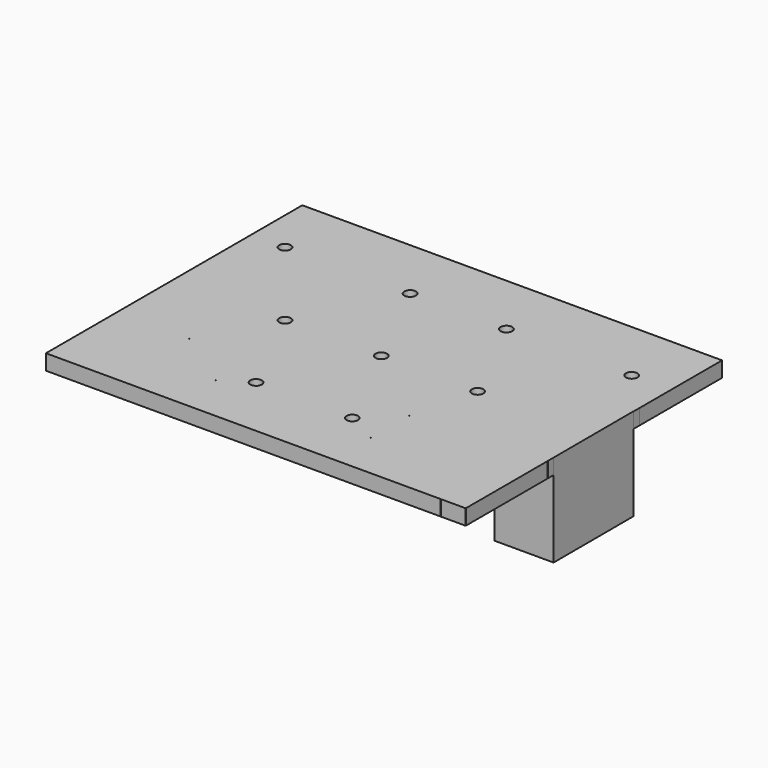
from build123d import *

# Parameters (mm, degrees)
F1_DEPTH = 2.54
F3_DEPTH = 12.7
F4_DEPTH = 2.54


# Not quite as in the source:
# - a feature names something its author has since deleted; it is built from what else it names


with BuildPart() as f1:
    # F0 (on Top) → F1 (new body)
    with BuildSketch(Plane.XY):
        with BuildLine():
            ThreePointArc((24.89835, -8.3058), (24.9076493597, -8.2833493597), (24.9301, -8.27405))
            Line((24.9301, -8.27405), (24.9301, 8.14705))
            ThreePointArc((24.9301, 8.14705), (24.9076493597, 8.1563493597), (24.89835, 8.1788))
            ThreePointArc((24.89835, 8.1788), (24.9301, 8.21055), (24.96185, 8.1788))
            Line((24.96185, 8.1788), (34.57575, 8.1788))
            ThreePointArc((34.57575, 8.1788), (34.5850493597, 8.2012506403), (34.6075, 8.21055))
            Line((34.6075, 8.21055), (34.6075, 9.36625))
            ThreePointArc((34.6075, 9.36625), (34.5850493597, 9.3755493597), (34.57575, 9.398))
            ThreePointArc((34.57575, 9.398), (34.5850493597, 9.4204506403), (34.6075, 9.42975))
            Line((34.6075, 9.42975), (34.6075, 26.38425))
            ThreePointArc((34.6075, 26.38425), (34.5850493597, 26.3935493597), (34.57575, 26.416))
            Line((34.57575, 26.416), (-34.57575, 26.416))
            ThreePointArc((-34.57575, 26.416), (-34.5850493597, 26.3935493597), (-34.6075, 26.38425))
            Line((-34.6075, 26.38425), (-34.6075, -26.38425))
            ThreePointArc((-34.6075, -26.38425), (-34.5850493597, -26.3935493597), (-34.57575, -26.416))
            Line((-34.57575, -26.416), (30.48635, -26.416))
            ThreePointArc((30.48635, -26.416), (30.5181, -26.38425), (30.54985, -26.416))
            Line((30.54985, -26.416), (34.57575, -26.416))
            ThreePointArc((34.57575, -26.416), (34.5850493597, -26.3935493597), (34.6075, -26.38425))
            Line((34.6075, -26.38425), (34.6075, -9.55675))
            ThreePointArc((34.6075, -9.55675), (34.5850493597, -9.5474506403), (34.57575, -9.525))
            ThreePointArc((34.57575, -9.525), (34.5850493597, -9.5025493597), (34.6075, -9.49325))
            Line((34.6075, -9.49325), (34.6075, -8.33755))
            ThreePointArc((34.6075, -8.33755), (34.5850493597, -8.3282506403), (34.57575, -8.3058))
            Line((34.57575, -8.3058), (24.96185, -8.3058))
            ThreePointArc((24.96185, -8.3058), (24.9301, -8.33755), (24.89835, -8.3058))
        make_face()
        with BuildLine():
            Line((-12.8397, -11.79195), (-12.8397, -18.61185))
            ThreePointArc((-12.8397, -18.61185), (-12.8172493597, -18.6211493597), (-12.80795, -18.6436))
            ThreePointArc((-12.80795, -18.6436), (-12.8397, -18.67535), (-12.87145, -18.6436))
            Line((-12.87145, -18.6436), (-22.68855, -18.6436))
            ThreePointArc((-22.68855, -18.6436), (-22.7203, -18.67535), (-22.75205, -18.6436))
            ThreePointArc((-22.75205, -18.6436), (-22.7427506403, -18.6211493597), (-22.7203, -18.61185))
            Line((-22.7203, -18.61185), (-22.7203, -11.79195))
            ThreePointArc((-22.7203, -11.79195), (-22.7427506403, -11.7826506403), (-22.75205, -11.7602))
            ThreePointArc((-22.75205, -11.7602), (-22.7203, -11.72845), (-22.68855, -11.7602))
            Line((-22.68855, -11.7602), (-12.87145, -11.7602))
            ThreePointArc((-12.87145, -11.7602), (-12.8397, -11.72845), (-12.80795, -11.7602))
            ThreePointArc((-12.80795, -11.7602), (-12.8172493597, -11.7826506403), (-12.8397, -11.79195))
        make_face(mode=Mode.SUBTRACT)
        with BuildLine():
            ThreePointArc((-12.21105, -24.6126), (-12.2017506403, -24.5901493597), (-12.1793, -24.58085))
            Line((-12.1793, -24.58085), (-12.1793, -20.91055))
            ThreePointArc((-12.1793, -20.91055), (-12.2017506403, -20.9012506403), (-12.21105, -20.8788))
            ThreePointArc((-12.21105, -20.8788), (-12.1793, -20.84705), (-12.14755, -20.8788))
            Line((-12.14755, -20.8788), (9.22655, -20.8788))
            ThreePointArc((9.22655, -20.8788), (9.2583, -20.84705), (9.29005, -20.8788))
            ThreePointArc((9.29005, -20.8788), (9.2807506403, -20.9012506403), (9.2583, -20.91055))
            Line((9.2583, -20.91055), (9.2583, -24.58085))
            ThreePointArc((9.2583, -24.58085), (9.2807506403, -24.5901493597), (9.29005, -24.6126))
            ThreePointArc((9.29005, -24.6126), (9.2583, -24.64435), (9.22655, -24.6126))
            Line((9.22655, -24.6126), (-12.14755, -24.6126))
            ThreePointArc((-12.14755, -24.6126), (-12.1793, -24.64435), (-12.21105, -24.6126))
        make_face(mode=Mode.SUBTRACT)
        with BuildLine():
            ThreePointArc((-7.4422, -15.875), (-8.3947, -16.8275), (-9.3472, -15.875))
            ThreePointArc((-9.3472, -15.875), (-8.3947, -14.9225), (-7.4422, -15.875))
        make_face(mode=Mode.SUBTRACT)
        with BuildLine():
            ThreePointArc((8.4328, -15.875), (7.4803, -16.8275), (6.5278, -15.875))
            ThreePointArc((6.5278, -15.875), (7.4803, -14.9225), (8.4328, -15.875))
        make_face(mode=Mode.SUBTRACT)
        with BuildLine():
            ThreePointArc((12.75715, -18.669), (12.7664493597, -18.6465493597), (12.7889, -18.63725))
            Line((12.7889, -18.63725), (12.7889, -10.82675))
            ThreePointArc((12.7889, -10.82675), (12.7664493597, -10.8174506403), (12.75715, -10.795))
            ThreePointArc((12.75715, -10.795), (12.7889, -10.76325), (12.82065, -10.795))
            Line((12.82065, -10.795), (18.90395, -10.795))
            ThreePointArc((18.90395, -10.795), (18.9357, -10.76325), (18.96745, -10.795))
            ThreePointArc((18.96745, -10.795), (18.9581506403, -10.8174506403), (18.9357, -10.82675))
            Line((18.9357, -10.82675), (18.9357, -18.63725))
            ThreePointArc((18.9357, -18.63725), (18.9581506403, -18.6465493597), (18.96745, -18.669))
            ThreePointArc((18.96745, -18.669), (18.9357, -18.70075), (18.90395, -18.669))
            Line((18.90395, -18.669), (12.82065, -18.669))
            ThreePointArc((12.82065, -18.669), (12.7889, -18.70075), (12.75715, -18.669))
        make_face(mode=Mode.SUBTRACT)
        with BuildLine():
            ThreePointArc((-15.367, 0), (-16.3195, -0.9525), (-17.272, 0))
            ThreePointArc((-17.272, 0), (-16.3195, 0.9525), (-15.367, 0))
        make_face(mode=Mode.SUBTRACT)
        with BuildLine():
            ThreePointArc((0.508, 0), (-0.4445, -0.9525), (-1.397, 0))
            ThreePointArc((-1.397, 0), (-0.4445, 0.9525), (0.508, 0))
        make_face(mode=Mode.SUBTRACT)
        with BuildLine():
            ThreePointArc((-28.067, 15.875), (-29.0195, 14.9225), (-29.972, 15.875))
            ThreePointArc((-29.972, 15.875), (-29.0195, 16.8275), (-28.067, 15.875))
        make_face(mode=Mode.SUBTRACT)
        with BuildLine():
            ThreePointArc((-7.4422, 15.875), (-8.3947, 14.9225), (-9.3472, 15.875))
            ThreePointArc((-9.3472, 15.875), (-8.3947, 16.8275), (-7.4422, 15.875))
        make_face(mode=Mode.SUBTRACT)
        with BuildLine():
            ThreePointArc((16.383, 0), (15.4305, -0.9525), (14.478, 0))
            ThreePointArc((14.478, 0), (15.4305, 0.9525), (16.383, 0))
        make_face(mode=Mode.SUBTRACT)
        with BuildLine():
            ThreePointArc((8.4328, 15.875), (7.4803, 14.9225), (6.5278, 15.875))
            ThreePointArc((6.5278, 15.875), (7.4803, 16.8275), (8.4328, 15.875))
        make_face(mode=Mode.SUBTRACT)
        with BuildLine():
            ThreePointArc((29.083, 15.875), (28.1305, 14.9225), (27.178, 15.875))
            ThreePointArc((27.178, 15.875), (28.1305, 16.8275), (29.083, 15.875))
        make_face(mode=Mode.SUBTRACT)
        with BuildLine():
            Line((12.7889, -10.82675), (12.7889, -18.63725))
            ThreePointArc((12.7889, -18.63725), (12.8113506403, -18.6465493597), (12.82065, -18.669))
            Line((12.82065, -18.669), (18.90395, -18.669))
            ThreePointArc((18.90395, -18.669), (18.9132493597, -18.6465493597), (18.9357, -18.63725))
            Line((18.9357, -18.63725), (18.9357, -10.82675))
            ThreePointArc((18.9357, -10.82675), (18.9132493597, -10.8174506403), (18.90395, -10.795))
            Line((18.90395, -10.795), (12.82065, -10.795))
            ThreePointArc((12.82065, -10.795), (12.8113506403, -10.8174506403), (12.7889, -10.82675))
        make_face()
        with BuildLine():
            Line((-12.1793, -20.91055), (-12.1793, -24.58085))
            ThreePointArc((-12.1793, -24.58085), (-12.1568493597, -24.5901493597), (-12.14755, -24.6126))
            Line((-12.14755, -24.6126), (9.22655, -24.6126))
            ThreePointArc((9.22655, -24.6126), (9.2358493597, -24.5901493597), (9.2583, -24.58085))
            Line((9.2583, -24.58085), (9.2583, -20.91055))
            ThreePointArc((9.2583, -20.91055), (9.2358493597, -20.9012506403), (9.22655, -20.8788))
            Line((9.22655, -20.8788), (-12.14755, -20.8788))
            ThreePointArc((-12.14755, -20.8788), (-12.1568493597, -20.9012506403), (-12.1793, -20.91055))
        make_face()
        with BuildLine():
            ThreePointArc((-12.87145, -18.6436), (-12.8621506403, -18.6211493597), (-12.8397, -18.61185))
            Line((-12.8397, -18.61185), (-12.8397, -11.79195))
            ThreePointArc((-12.8397, -11.79195), (-12.8621506403, -11.7826506403), (-12.87145, -11.7602))
            Line((-12.87145, -11.7602), (-22.68855, -11.7602))
            ThreePointArc((-22.68855, -11.7602), (-22.6978493597, -11.7826506403), (-22.7203, -11.79195))
            Line((-22.7203, -11.79195), (-22.7203, -18.61185))
            ThreePointArc((-22.7203, -18.61185), (-22.6978493597, -18.6211493597), (-22.68855, -18.6436))
            Line((-22.68855, -18.6436), (-12.87145, -18.6436))
        make_face()
    extrude(amount=F1_DEPTH)

    # F2 (on face) → F3 (join)
    with BuildSketch(Plane(origin=(0, 0, 0), x_dir=(1, 0, 0), z_dir=(0, 0, -1))):
        with BuildLine():
            Line((24.96185, -8.1788), (34.57575, -8.1788))
            Line((34.57575, -8.1788), (34.6075, 8.33755))
            ThreePointArc((34.6075, 8.33755), (34.5850493597, 8.3282506403), (34.57575, 8.3058))
            Line((34.57575, 8.3058), (24.96185, 8.3058))
            ThreePointArc((24.96185, 8.3058), (24.9076493597, 8.3282506403), (24.9301, 8.27405))
            Line((24.9301, 8.27405), (24.9301, -8.14705))
            ThreePointArc((24.9301, -8.14705), (24.9076493597, -8.2012506403), (24.96185, -8.1788))
        make_face()
    extrude(amount=F3_DEPTH)

    # F4 (add): a face of the model
    f4_faces = [f1.faces().sort_by_distance(p)[0] for p in [
        (29.7607313536, -0.0680465181, 0),
    ]]
    extrude(f4_faces, amount=F4_DEPTH)


solid = f1.part
